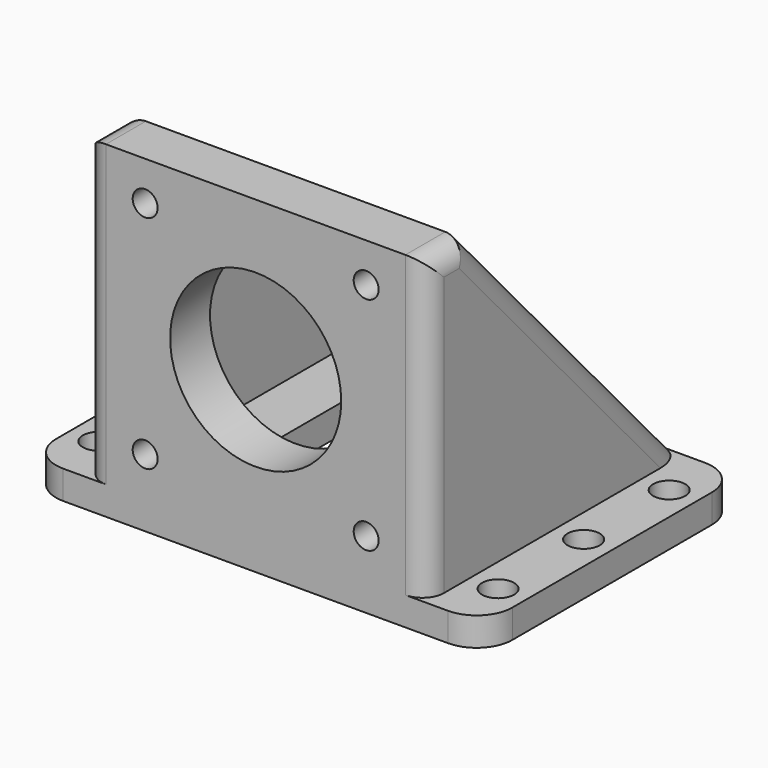
from build123d import *

# Parameters (mm, degrees)
F0_W      = 42
F0_H      = 42
F0_R      = 1.75
F0_R_2    = 12
F1_DEPTH  = 7
F0_W_2    = 3
F2_DEPTH  = 45
F3_DEPTH  = 45
F4_SIZE2  = 38
F4_SIZE   = 42
F5_R      = 2.25
F6_DEPTH  = 25
F7_R      = 5
F8_R      = 2.99999
F9_W      = 26
F9_H      = 22
F10_DEPTH = 25
F11_R     = 5


# Not quite as in the source:
# - a fillet or chamfer is up to 0.001 mm smaller than in the source, because OpenCascade refuses the exact size


with BuildPart() as f1:
    # F0 (on Front) → F1 (new body)
    with BuildSketch(Plane.XZ):
        Rectangle(F0_W, F0_H)
        with Locations((-15.5, -15.5)):
            Circle(F0_R, mode=Mode.SUBTRACT)
        with Locations((15.5, -15.5)):
            Circle(F0_R, mode=Mode.SUBTRACT)
        with Locations((-15.5, 15.5)):
            Circle(F0_R, mode=Mode.SUBTRACT)
        Circle(F0_R_2, mode=Mode.SUBTRACT)
        with Locations((15.5, 15.5)):
            Circle(F0_R, mode=Mode.SUBTRACT)
    extrude(amount=-F1_DEPTH)

    # F0 (on Front) → F2 (join)
    with BuildSketch(Plane.XZ):
        with Locations((22.5, 0)):
            Rectangle(F0_W_2, F0_H)
        with Locations((-22.5, 0)):
            Rectangle(F0_W_2, F0_H)
    extrude(amount=-F2_DEPTH)

    # F0 (on Front) → F3 (join, through all)
    with BuildSketch(Plane.XZ):
        Polygon((24, -21), (21, -21), (-21, -21), (-24, -21), (-32, -21), (-32, -25), (32, -25), (32, -21), align=None)
    extrude(amount=-F3_DEPTH)

    # F4
    f4_edges = [f1.edges().sort_by_distance(p)[0] for p in [
        (22.5, 45, 21),
        (-22.5, 45, 21),
    ]]
    f4_side = f1.faces().sort_by_distance((-31.211838, 45, -23))[0]
    chamfer(f4_edges, length=F4_SIZE, length2=F4_SIZE2, reference=f4_side)

    # F5 (on face) → F6 (cut)
    with BuildSketch(Plane.XY.offset(-21)):
        with Locations((28, 7.5)):
            Circle(F5_R)
        with Locations((28, 22.5)):
            Circle(F5_R)
        with Locations((28, 37.5)):
            Circle(F5_R)
        with Locations((-28, 7.5)):
            Circle(F5_R)
        with Locations((-28, 22.5)):
            Circle(F5_R)
        with Locations((-28, 37.5)):
            Circle(F5_R)
    extrude(amount=-F6_DEPTH, mode=Mode.SUBTRACT)

    # F7
    f7_edges = [f1.edges().sort_by_distance(p)[0] for p in [
        (-32, 0, -23),
        (-32, 45, -23),
        (32, 0, -23),
        (32, 45, -23),
    ]]
    fillet(f7_edges, radius=F7_R)

    # F8 (radius 3 in the source; OpenCascade refuses exactly that, so slightly less here)
    f8_edges = [f1.edges().sort_by_distance(p)[0] for p in [
        (24, 0, 0),
        (-24, 0, 0),
        (-24, 26, 0),
        (-24, 3.5, 21),
        (24, 3.5, 21),
        (24, 26, 0),
    ]]
    fillet(f8_edges, radius=F8_R)

    # F9 (on face) → F10 (cut)
    with BuildSketch(Plane.XY.offset(-21)):
        with Locations((0, 26)):
            Rectangle(F9_W, F9_H)
    extrude(amount=-F10_DEPTH, mode=Mode.SUBTRACT)

    # F11
    f11_edges = [f1.edges().sort_by_distance(p)[0] for p in [
        (13, 15, -23),
        (-13, 15, -23),
        (-13, 37, -23),
        (13, 37, -23),
    ]]
    fillet(f11_edges, radius=F11_R)


solid = f1.part
